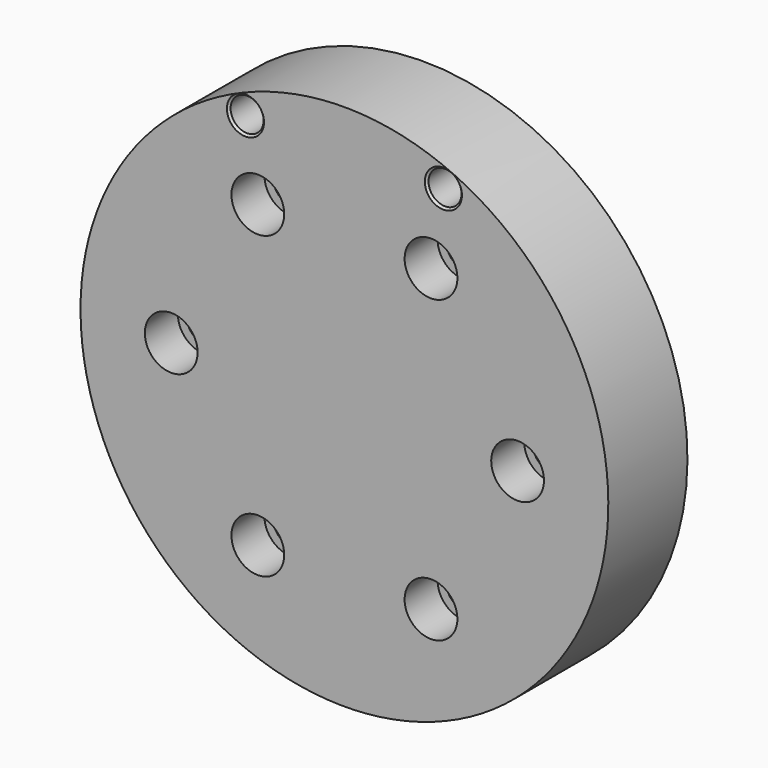
from build123d import *

# Parameters (mm, degrees)
F0_R           = 101.6
F1_DEPTH       = 38.1
F2_D           = 13.462
F2_DEPTH       = 50.8
F2_CBORE_D     = 20.32
F2_CBORE_DEPTH = 15.875
F2_TIP         = 4.0443928267
F3_D           = 13.462
F3_DEPTH       = 50.8
F3_CBORE_D     = 20.32
F3_CBORE_DEPTH = 15.875
F3_TIP         = 4.0443928267
F4_ANGLE       = 30
F6_D           = 12.7
F6_DEPTH       = 50.8
F6_CSINK_D     = 14.2875
F6_CSINK_ANGLE = 90
F6_TIP         = 3.8154649308


# Not quite as in the source:
# - a feature names something its author has since deleted; it is built from what else it names


with BuildPart() as f1:
    # F0 (on Front) → F1 (new body)
    with BuildSketch(Plane.XZ):
        Circle(F0_R)
    extrude(amount=-F1_DEPTH)

    # F2
    with Locations(Plane.XZ):
        with Locations((0, 66.675)):
            CounterBoreHole(F2_D / 2, F2_CBORE_D / 2, F2_CBORE_DEPTH, depth=F2_DEPTH)
            with Locations((0, 0, -(F2_DEPTH + F2_TIP / 2))):  # 118° drill point
                Cone(0, F2_D / 2, F2_TIP, mode=Mode.SUBTRACT)

    # F3
    with Locations(Plane.XZ):
        with Locations((-57.7422437973, 33.3375), (-57.7422437973, -33.3375), (0, -66.675), (57.7422437973, -33.3375), (57.7422437973, 33.3375)):
            CounterBoreHole(F3_D / 2, F3_CBORE_D / 2, F3_CBORE_DEPTH, depth=F3_DEPTH)
            with Locations((0, 0, -(F3_DEPTH + F3_TIP / 2))):  # 118° drill point
                Cone(0, F3_D / 2, F3_TIP, mode=Mode.SUBTRACT)


with BuildPart() as f1_1:
    # F4: moved
    add(f1.part.rotate(Axis((0, 0, 0), (0, -1, 0)), F4_ANGLE))


with BuildPart() as f1_2:
    # F5: moved
    add(f1_1.part.moved(Location((-846.1338678, 0, -154.2352516))))

    # F6
    with Locations(Plane.XZ):
        with Locations((-884.2338678, -67.8752516), (-808.0338678, -67.8752516)):
            CounterSinkHole(F6_D / 2, F6_CSINK_D / 2, depth=F6_DEPTH, counter_sink_angle=F6_CSINK_ANGLE)
            with Locations((0, 0, -(F6_DEPTH + F6_TIP / 2))):  # 118° drill point
                Cone(0, F6_D / 2, F6_TIP, mode=Mode.SUBTRACT)


solid = f1_2.part
